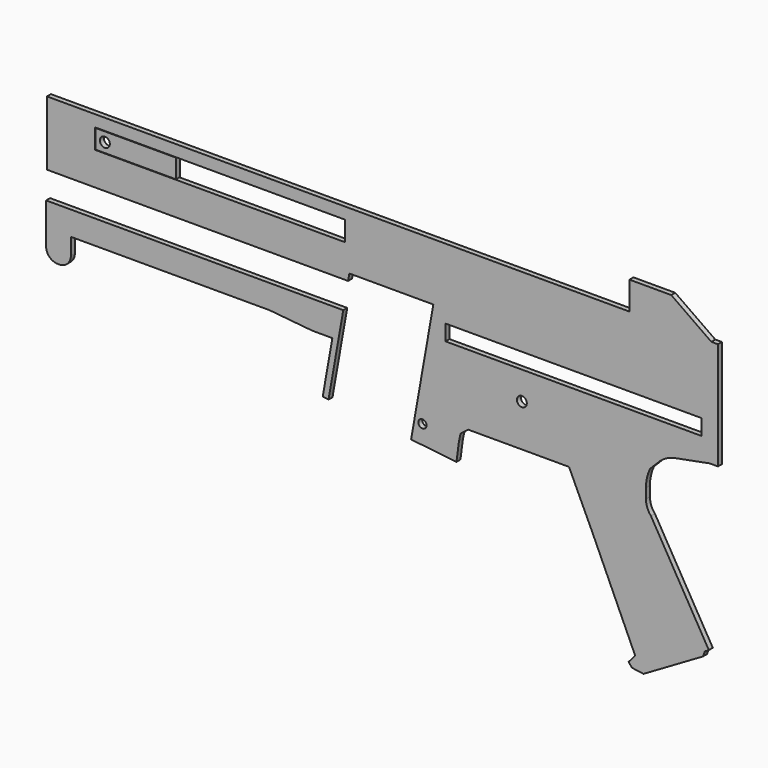
from build123d import *

# Parameters (mm, degrees)
F0_R     = 2.5
F0_W     = 151
F0_H     = 12
F0_R_2   = 3
F0_W_2   = 154.629
F0_H_2   = 9.5
F1_DEPTH = 3
F0_W_3   = 48.75
F0_H_3   = 11.5


# Not quite as in the source:
# - a feature names something its author has since deleted; it is built from what else it names


with BuildPart() as f1:
    # F0 (on Front) → F1 (new body)
    with BuildSketch(Plane.XZ):
        with BuildLine():
            Line((48.5, -65), (53.5, -65))
            Line((53.5, -65), (53.5, 0))
            Line((53.5, 0), (49.5, 0))
            Line((49.5, 0), (25.275, 17))
            Line((25.275, 17), (0, 17))
            Line((0, 17), (0, 0))
            Line((0, 0), (-352, 0))
            Line((-352, 0), (-352, -39))
            Line((-352, -39), (-170.0255081496, -39))
            Line((-170.0255081496, -39), (-169.2796367248, -34.7699529486))
            Line((-169.2796367248, -34.7699529486), (-118.5083061305, -34.7699529486))
            Line((-118.5083061305, -34.7699529486), (-119.2130711177, -38.7668738074))
            Line((-119.2130711177, -38.7668738074), (-121.5464283045, -52))
            Line((-121.5464283045, -52), (-131.9409607911, -110.9503231145))
            Line((-131.9409607911, -110.9503231145), (-104.5337054221, -114))
            Line((-104.5337054221, -114), (-103, -102.5))
            Line((-103, -102.5), (-102, -98))
            Line((-102, -98), (-97.5, -94.5))
            Line((-97.5, -94.5), (-36.5, -94.5))
            Line((-36.5, -94.5), (-22.5, -124.5))
            Line((-22.5, -124.5), (3.5, -182))
            Line((3.5, -182), (-0.5, -186.5))
            Line((-0.5, -186.5), (1.5, -189))
            Line((1.5, -189), (8.5, -190))
            Line((8.5, -190), (44.5, -169))
            Line((44.5, -169), (45.5, -166))
            Line((45.5, -166), (48, -164.5))
            Line((48, -164.5), (13, -104.5))
            ThreePointArc((13, -104.5), (10.7746616729, -100.7720018727), (10, -96.5))
            Line((10, -96.5), (10, -90.5))
            ThreePointArc((10, -90.5), (10.6328688201, -84.8597429137), (12.5, -79.5))
            Line((12.5, -79.5), (18.5, -73.5))
            ThreePointArc((18.5, -73.5), (22.688171875, -70.6263437501), (27.5, -69))
            Line((27.5, -69), (48.5, -65))
        make_face()
        with Locations((-125.101, -100.41)):
            Circle(F0_R, mode=Mode.SUBTRACT)
        with Locations((-247.5, -13)):
            Rectangle(F0_W, F0_H, mode=Mode.SUBTRACT)
        with Locations((-65, -69)):
            Circle(F0_R_2, mode=Mode.SUBTRACT)
        with Locations((-33.8145, -47.25)):
            Rectangle(F0_W_2, F0_H_2, mode=Mode.SUBTRACT)
    extrude(amount=F1_DEPTH)


with BuildPart() as f1b:
    # F0 (on Front) → F1, piece 2 (new body)
    with BuildSketch(Plane.XZ):
        with BuildLine():
            ThreePointArc((-352.5206254937, -80), (-350.470372962, -84.9497474683), (-345.5206254937, -87))
            Line((-345.5206254937, -87), (-344.5206254937, -87))
            ThreePointArc((-344.5206254937, -87), (-339.5708780254, -84.9497474683), (-337.5206254937, -80))
            Line((-337.5206254937, -80), (-337.5206254937, -70))
            Line((-337.5206254937, -70), (-217.5206254937, -70))
            Line((-217.5206254937, -70), (-191.5206254937, -72.5))
            Line((-191.5206254937, -72.5), (-179.5206254937, -72.5))
            Line((-179.5206254937, -72.5), (-185.3394158571, -105.5))
            Line((-185.3394158571, -105.5), (-181.8394158571, -106))
            Line((-181.8394158571, -106), (-172.9349033313, -55.5))
            Line((-172.9349033313, -55.5), (-352.5206254937, -55.5))
            Line((-352.5206254937, -55.5), (-352.5206254937, -80))
        make_face()
    extrude(amount=F1_DEPTH)


with BuildPart() as f1c:
    # F0 (on Front) → F1, piece 3 (new body)
    with BuildSketch(Plane.XZ):
        with Locations((-298.375, -13)):
            Rectangle(F0_W_3, F0_H_3)
        with Locations((-317, -13)):
            Circle(F0_R_2, mode=Mode.SUBTRACT)
    extrude(amount=F1_DEPTH)


solid = Compound([f1.part, f1b.part, f1c.part])
